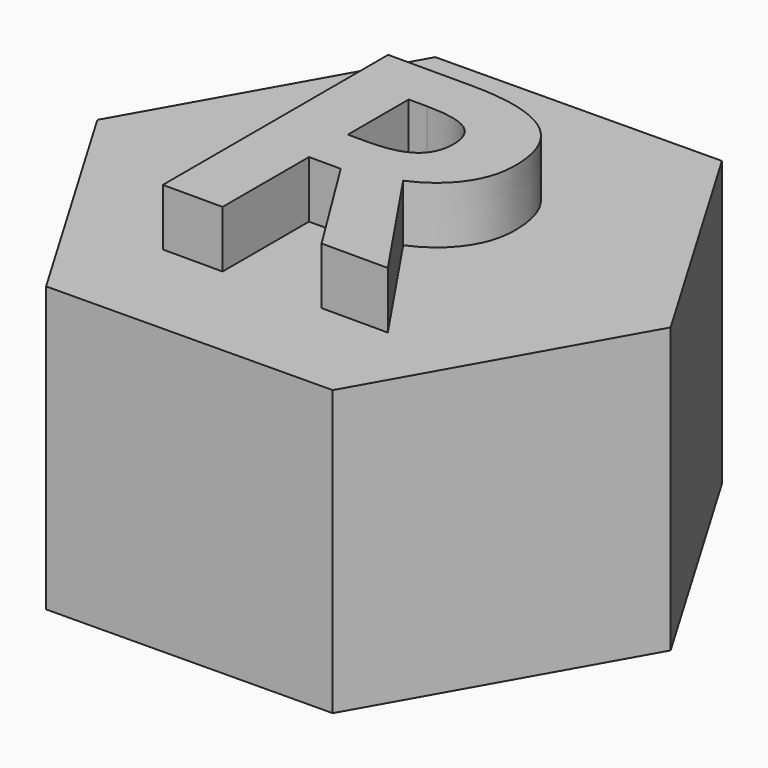
from build123d import *

# Parameters (mm, degrees)
F1_DEPTH     = 12.7
F2_TEXT_SIZE = 17.6147273224
F3_DEPTH     = 2.54


# Not quite as in the source:
# - Text() gives the source's letters only with a copy of the font that has no kerning and outlines rounded to 1/6400 em; it was checked with that copy


with BuildPart() as f1:
    # F0 (on Top) → F1 (new body)
    with BuildSketch(Plane.XY):
        Polygon((12.6993846473, 0.1250183213), (6.2414232815, 11.0604988776), (-6.4579613658, 10.9354805563), (-12.6993846473, -0.1250183213), (-6.2414232815, -11.0604988776), (6.4579613658, -10.9354805563), align=None)
    extrude(amount=F1_DEPTH)

    # F2 (on face) → F3 (join)
    with BuildSketch(Plane.XY.offset(12.7)):
        with Locations((-6.3853386544, -6.3413018361)):
            Text('R', F2_TEXT_SIZE, font='Open Sans', font_style=FontStyle.BOLD, text_align=(TextAlign.LEFT, TextAlign.BOTTOM))
    extrude(amount=F3_DEPTH)


solid = f1.part
